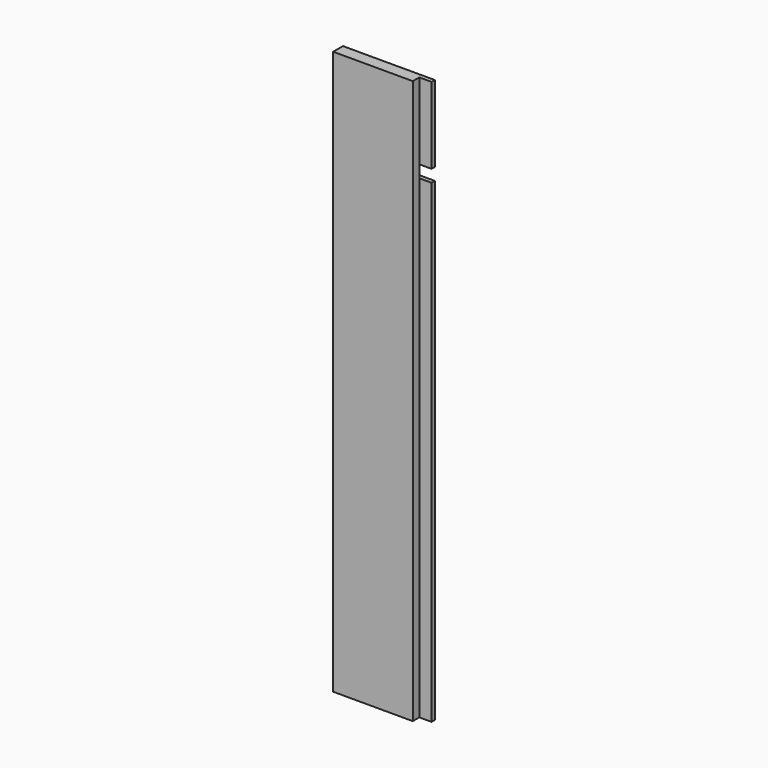
from build123d import *

# Parameters (mm, degrees)
F0_W     = 142.875
F0_H     = 438.15
F1_DEPTH = 9.525
F2_W     = 142.875
F2_H     = 19.05
F3_DEPTH = 6.35
F4_W     = 19.05
F4_H     = 876.3
F5_DEPTH = 12.7


# Not quite as in the source:
# - a feature names something its author has since deleted; it is built from what else it names


with BuildPart() as f1:
    # F0 (on Front) → F1 (new body, symmetric)
    with BuildSketch(Plane.XZ):
        with Locations((-176.4664953259, 219.075)):
            Rectangle(F0_W, F0_H)
        with Locations((-176.4664953259, -219.075)):
            Rectangle(F0_W, F0_H)
    extrude(amount=F1_DEPTH, both=True)

    # F2 (on face) → F3 (cut)
    with BuildSketch(Plane(origin=(0, 9.525, 0), x_dir=(-1, 0, 0), z_dir=(0, 1, 0))):
        with Locations((176.4664953259, 309.5625)):
            Rectangle(F2_W, F2_H)
    extrude(amount=-F3_DEPTH, mode=Mode.SUBTRACT)

    # F4 (on face) → F5 (cut)
    with BuildSketch(Plane.XZ.offset(9.525)):
        with Locations((-114.5539953259, 0)):
            Rectangle(F4_W, F4_H)
    extrude(amount=-F5_DEPTH, mode=Mode.SUBTRACT)


solid = f1.part
